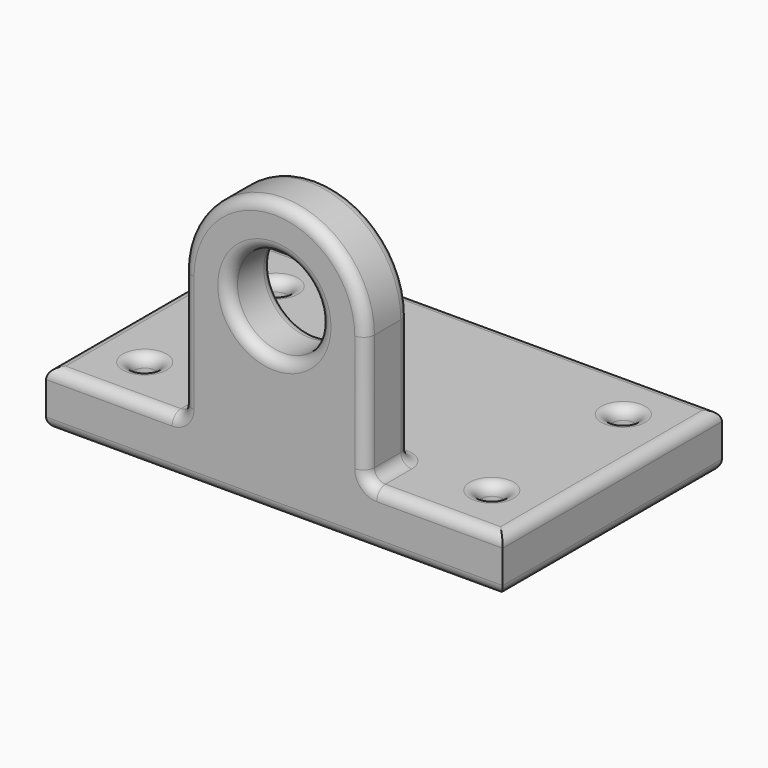
from build123d import *

# Parameters (mm, degrees)
F0_W     = 125
F0_H     = 75
F0_R     = 3
F1_DEPTH = 15
F2_W     = 50
F2_H     = 15
F3_DEPTH = 15
F4_R     = 3


with BuildPart() as f1:
    # F0 (on Top) → F1 (new body)
    with BuildSketch(Plane.XY):
        Rectangle(F0_W, F0_H)
        with Locations((-47.5, -22.5)):
            Circle(F0_R, mode=Mode.SUBTRACT)
        with Locations((47.5, -22.5)):
            Circle(F0_R, mode=Mode.SUBTRACT)
        with Locations((-47.5, 22.5)):
            Circle(F0_R, mode=Mode.SUBTRACT)
        with Locations((47.5, 22.5)):
            Circle(F0_R, mode=Mode.SUBTRACT)
    extrude(amount=F1_DEPTH)

    # F2 (on face) → F3 (join)
    with BuildSketch(Plane.XZ.offset(37.5)):
        with BuildLine():
            Line((12.5, 50), (25, 50))
            ThreePointArc((25, 50), (0, 75), (-25, 50))
            Line((-25, 50), (-12.5, 50))
            ThreePointArc((-12.5, 50), (0, 62.5), (12.5, 50))
        make_face()
        with BuildLine():
            ThreePointArc((-25, 50), (0, 25), (25, 50))
            Line((25, 50), (12.5, 50))
            ThreePointArc((12.5, 50), (0, 37.5), (-12.5, 50))
            Line((-12.5, 50), (-25, 50))
        make_face()
        with BuildLine():
            Line((25, 15), (25, 50))
            ThreePointArc((25, 50), (0, 25), (-25, 50))
            Line((-25, 50), (-25, 15))
            Line((-25, 15), (25, 15))
        make_face()
        with Locations((0, 7.5)):
            Rectangle(F2_W, F2_H)
    extrude(amount=-F3_DEPTH)

    # F4
    f4_edges = [f1.edges().sort_by_distance(p)[0] for p in [
        (43.75, -37.5, 15),
        (25, -30, 15),
        (0, -22.5, 15),
        (-25, -30, 15),
        (-43.75, -37.5, 15),
        (-62.5, 0, 15),
        (0, 37.5, 15),
        (62.5, 0, 15),
        (-50.5, -22.5, 15),
        (44.5, -22.5, 15),
        (-50.5, 22.5, 15),
        (44.5, 22.5, 15),
        (25, -22.5, 32.5),
        (-25, -22.5, 32.5),
        (0, -22.5, 75),
        (-12.5, -22.5, 50),
        (-12.5, -37.5, 50),
        (62.5, 0, 0),
        (0, 37.5, 0),
        (-62.5, 0, 0),
        (0, -37.5, 0),
        (-50.5, -22.5, 0),
        (44.5, -22.5, 0),
        (-50.5, 22.5, 0),
        (44.5, 22.5, 0),
        (-25, -37.5, 32.5),
        (0, -37.5, 75),
        (25, -37.5, 32.5),
    ]]
    fillet(f4_edges, radius=F4_R)


solid = f1.part
